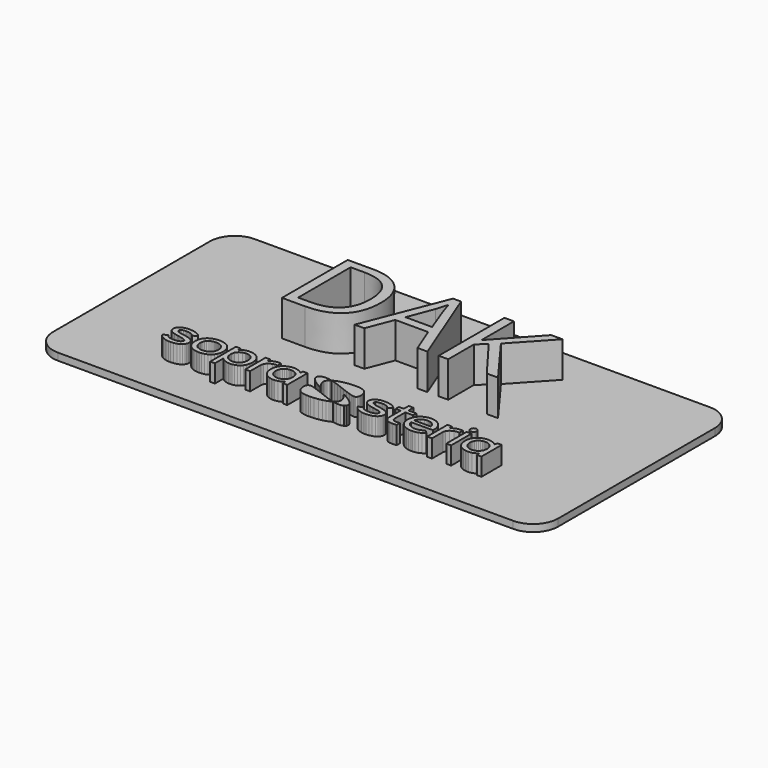
from build123d import *

# Parameters (mm, degrees)
F1_DEPTH     = 12.7
F0_W         = 3.439668
F0_H         = 17.9889404
F2_TEXT_SIZE = 81.8710528274
F3_DEPTH     = 25.4
F5_DEPTH     = 5.08


# Not quite as in the source:
# - Text() gives the source's letters only with a copy of the font that has no kerning and outlines rounded to 1/6400 em; it was checked with that copy


with BuildPart() as f1:
    # F0 (on Top) → F1 (new body)
    with BuildSketch(Plane.XY):
        Polygon((10.402189, -8.9867994), (10.078339, -9.2017596), (10.030333, -9.2320872), (9.500997, -9.561449), (9.448419, -9.5917512), (9.3881075175, -9.6273787491), (9.389237, -9.6275906), (9.38663303, -9.629093988), (9.448419, -9.6358456), (10.190099, -9.8384106), (12.472035, -10.2407974), (15.177135, -10.2821486), (17.257903, -9.6289622), (18.283047, -8.5747606), (18.410047, -8.1585816), (18.496915, -7.8691994), (18.455513, -6.9086222), (17.923637, -5.6614822), (16.941165, -4.4420282), (15.638653, -3.2733742), (14.143609, -2.1806662), (12.585065, -1.1885422), (11.092561, -0.3203702), (10.119741, 0.2186178), (9.795891, 0.3961638), (9.696577, 0.4500118), (9.375521, 0.5630418), (9.126093, 0.5409438), (9.080627, 0.3590798), (9.209913, 0.1152398), (9.269349, 0.0476758), (9.465183, -0.1783842), (10.023221, -0.8867902), (10.767441, -1.9794982), (11.413871, -3.1811722), (11.872341, -4.4460922), (12.055983, -5.7262522), (11.876659, -6.9777102), (11.246993, -8.1517236), align=None)
        Polygon((9.389237, -9.6275906), (9.3881075175, -9.6273787491), (9.385427, -9.6289622), (9.38663303, -9.629093988), align=None)
        Polygon((9.385427, -9.6289622), (9.3881075175, -9.6273787491), (8.749919, -9.5076772), (6.863461, -8.988171), (3.947541, -8.0138778), (0.805561, -6.8342002), (-2.398395, -5.5789322), (-5.497703, -4.3757342), (-8.328025, -3.3561782), (-10.724515, -2.6492962), (-12.073763, -2.3858982), (-12.522835, -2.3858982), (-12.767945, -2.3858982), (-13.502513, -2.6396442), (-14.194409, -3.3300162), (-14.606397, -4.3442382), (-14.741525, -5.2660042), (-14.741525, -5.5733442), (-14.741525, -5.9563762), (-14.609191, -7.1057262), (-14.216507, -8.6050628), (-13.575665, -9.9693222), (-12.948539, -10.8498894), (-12.695047, -11.0993174), (-12.437491, -11.3528856), (-11.446637, -11.8999762), (-9.662287, -12.4539502), (-7.450201, -12.7750062), (-5.552567, -12.8797558), (-4.918837, -12.8797558), (-4.109847, -12.8797558), (-1.681861, -12.7391922), (1.169543, -12.3712478), (3.620897, -11.8503446), (5.660263, -11.2536478), (7.269861, -10.6555794), (8.436991, -10.1347016), (9.148191, -9.7667572), (9.38663303, -9.629093988), align=None)
    extrude(amount=F1_DEPTH)


with BuildPart() as f1b:
    # F0 (on Top) → F1, piece 2 (new body)
    with BuildSketch(Plane.XY):
        Polygon((42.048811, 5.3156358), (45.511847, 5.3156358), (45.511847, -3.8108382), (45.511847, -4.0231822), (45.539533, -4.6640242), (45.657897, -5.6147462), (45.919771, -6.5959482), (46.377225, -7.5438762), (47.082837, -8.3956144), (48.087661, -9.0832686), (49.446053, -9.5435166), (50.768885, -9.7116138), (51.210083, -9.7116138), (51.641375, -9.7116138), (52.938299, -9.6454722), (54.256813, -9.4994222), (54.548913, -9.4608396), (54.548913, -6.4387222), (54.343681, -6.4857122), (53.813075, -6.5918842), (53.082825, -6.6965322), (52.477797, -6.7447922), (52.276883, -6.7447922), (51.848131, -6.7447922), (50.562383, -6.5311782), (49.521999, -5.8987182), (49.006633, -4.8568102), (48.868711, -3.7750242), (48.868711, -3.4153602), (48.868711, 5.3156358), (54.393465, 5.3156358), (54.393465, 8.2165698), (48.868711, 8.2165698), (48.868711, 12.5172978), (45.511847, 12.5172978), (45.511847, 8.2165698), (42.048811, 8.2165698), align=None)
    extrude(amount=F1_DEPTH)


with BuildPart() as f1c:
    # F0 (on Top) → F1, piece 3 (new body)
    with BuildSketch(Plane.XY):
        with Locations((91.832049, -0.7598664)):
            Rectangle(F0_W, F0_H)
    extrude(amount=F1_DEPTH)


with BuildPart() as f1d:
    # F0 (on Top) → F1, piece 4 (new body)
    with BuildSketch(Plane.XY):
        Polygon((96.128459, -0.0089662), (96.128459, -0.5918962), (96.128459, -1.1705082), (96.347661, -2.9096462), (96.963611, -4.8555402), (97.911793, -6.4471042), (99.127183, -7.7051916), (100.543741, -8.6491572), (102.096697, -9.2982288), (103.723059, -9.6730566), (104.947847, -9.7943162), (105.357041, -9.7943162), (106.061637, -9.7943162), (108.174155, -9.42086), (110.188883, -8.600948), (111.398431, -7.7810106), (111.802291, -7.4090022), (111.976027, -9.790176), (115.120547, -9.790176), (115.120547, 8.2330798), (111.981615, 8.2330798), (111.802291, 5.9966098), (111.406813, 6.3839598), (110.216315, 7.2340978), (108.216827, 8.0842358), (106.099991, 8.4703158), (105.395903, 8.4703158), (105.022269, 8.4703158), (103.906193, 8.3585558), (102.344855, 8.0057498), (100.793169, 7.3872598), (99.336733, 6.4759078), (98.057843, 5.2483258), (97.042097, 3.6788598), (96.369759, 1.7398238), align=None)
        Polygon((99.623499, -1.0437622), (99.623499, -0.6277102), (99.623499, -0.2045462), (99.799775, 1.0631678), (100.280597, 2.4246078), (100.995861, 3.4873438), (101.872415, 4.2838878), (102.835583, 4.8485298), (103.816531, 5.2112418), (104.741091, 5.4052978), (105.339515, 5.4616858), (105.539159, 5.4616858), (106.134535, 5.4616858), (107.923203, 5.1022758), (109.919897, 4.0011858), (111.292513, 2.1256498), (111.802291, 0.1137158), (111.802291, -0.5573522), (111.802291, -1.2340082), (111.342043, -3.2652462), (110.056549, -5.1999642), (108.087287, -6.3617602), (106.202099, -6.7488562), (105.575227, -6.7488562), (105.372281, -6.7488562), (104.768777, -6.6853562), (103.837359, -6.4813942), (102.850569, -6.1039502), (101.880543, -5.5250842), (101.001449, -4.7176182), (100.283391, -3.6510722), (99.799775, -2.2964902), align=None, mode=Mode.SUBTRACT)
    extrude(amount=F1_DEPTH)


with BuildPart() as f1e:
    # F0 (on Top) → F1, piece 5 (new body)
    with BuildSketch(Plane.XY):
        Polygon((94.080965, 12.1688098), (94.080965, 12.3864878), (94.080965, 12.6054358), (93.903165, 13.2630418), (93.420819, 13.9767818), (92.706825, 14.4591278), (92.049727, 14.6354038), (91.832049, 14.6354038), (91.612847, 14.6354038), (90.955241, 14.4591278), (90.241755, 13.9767818), (89.759409, 13.2630418), (89.583133, 12.6054358), (89.583133, 12.3864878), (89.583133, 12.1688098), (89.759409, 11.5114578), (90.241755, 10.7964478), (90.955241, 10.3153718), (91.612847, 10.1375718), (91.832049, 10.1375718), (92.049727, 10.1375718), (92.706825, 10.3153718), (93.420819, 10.7964478), (93.903165, 11.5114578), align=None)
    extrude(amount=F1_DEPTH)


with BuildPart() as f1f:
    # F0 (on Top) → F1, piece 6 (new body)
    with BuildSketch(Plane.XY):
        Polygon((86.724871, 5.1904138), (87.600155, 5.1406298), (87.600155, 8.1876138), (87.012653, 8.2412078), (85.235161, 8.2099658), (83.205193, 7.8101698), (81.461991, 6.9889878), (80.297655, 6.0943998), (79.964153, 5.7443878), (79.785083, 8.2252058), (76.524739, 8.2252058), (76.524739, -9.7777808), (79.964153, -9.7777808), (79.964153, -0.4499102), (79.964153, 0.0545338), (80.377665, 1.5663418), (81.704815, 3.4388298), (84.069555, 4.7647098), align=None)
    extrude(amount=F1_DEPTH)


with BuildPart() as f1g:
    # F0 (on Top) → F1, piece 7 (new body)
    with BuildSketch(Plane.XY):
        Polygon((55.218711, -0.1562862), (55.218711, -0.6607302), (55.218711, -0.7999222), (55.218711, -1.2903962), (55.409211, -2.7620722), (55.965725, -4.5245782), (56.861583, -6.0681362), (58.067321, -7.3716642), (59.556777, -8.4190586), (61.304043, -9.1907614), (63.281687, -9.6661478), (64.917447, -9.8301556), (65.463293, -9.8301556), (66.000503, -9.8301556), (67.612641, -9.6785684), (69.688075, -9.1659456), (71.684769, -8.204073), (73.162287, -7.1222362), (73.598913, -6.7046602), (71.139177, -4.5413422), (70.752081, -4.8857662), (69.636005, -5.6437022), (67.851147, -6.4016382), (66.058415, -6.7475862), (65.461769, -6.7475862), (64.856741, -6.7475862), (63.043181, -6.3754762), (60.941585, -5.3516022), (59.432825, -3.8067742), (58.820939, -2.3625302), (58.796047, -1.8733262), (74.168127, -1.8085562), (74.186161, -1.6350742), (74.231627, -0.8177022), (74.241025, -0.3493262), (74.241025, 0.0984758), (74.066019, 1.4408658), (73.562083, 3.1121858), (72.750299, 4.6295818), (71.655813, 5.9524138), (70.301231, 7.0468998), (68.713731, 7.8746858), (66.915665, 8.3986878), (65.427225, 8.5802978), (64.932687, 8.5802978), (64.428243, 8.5802978), (62.919483, 8.4151978), (61.071125, 7.9287878), (59.417839, 7.1416418), (57.991375, 6.0710318), (56.826785, 4.7372778), (55.954549, 3.1576518), (55.407687, 1.3527278), align=None)
        Polygon((70.465315, 1.1086338), (70.465315, 0.8840978), (58.848625, 0.8840978), (58.887233, 1.3318998), (59.442477, 2.6341578), (60.780549, 4.0590978), (62.685041, 5.0184558), (64.404875, 5.3682138), (64.979169, 5.3682138), (65.255013, 5.3682138), (66.083053, 5.2757578), (67.112515, 5.0126138), (68.044187, 4.5950378), (68.855971, 4.0438578), (69.526785, 3.3783778), (70.032753, 2.6176478), (70.352539, 1.7799558), align=None, mode=Mode.SUBTRACT)
    extrude(amount=F1_DEPTH)


with BuildPart() as f1h:
    # F0 (on Top) → F1, piece 8 (new body)
    with BuildSketch(Plane.XY):
        Polygon((35.330765, 0.8454898), (34.687383, 0.9597898), (34.053399, 1.0728198), (32.153225, 1.4103858), (29.956633, 1.9188938), (28.407487, 2.6148538), (27.821763, 3.3730438), (27.821763, 3.6247578), (27.821763, 3.8139878), (28.031313, 4.3773598), (28.721939, 5.0085498), (29.979747, 5.4413658), (31.415863, 5.6011318), (31.895415, 5.6011318), (32.323913, 5.6011318), (33.613725, 5.4949598), (35.252533, 5.1421538), (36.600003, 4.4891198), (37.320855, 3.7738558), (37.448871, 3.4845498), (40.640381, 4.8254158), (40.414575, 5.2800758), (39.305103, 6.4281558), (37.246433, 7.5622658), (34.639377, 8.2361278), (32.402653, 8.4578698), (31.656909, 8.4578698), (30.979237, 8.4578698), (28.949269, 8.1863438), (26.533475, 7.3128378), (24.797131, 5.7499758), (24.132921, 3.9955978), (24.132921, 3.4101278), (24.132921, 2.9084778), (24.659209, 1.4022578), (26.176605, 0.0199898), (28.589605, -0.9335262), (30.993969, -1.5055342), (31.802959, -1.6584422), (32.377761, -1.7658842), (34.105977, -2.0800822), (36.065333, -2.5512522), (37.425503, -3.2322262), (37.935281, -4.0203882), (37.935281, -4.2835322), (37.935281, -4.4943522), (37.651563, -5.1268122), (36.758499, -5.9276742), (35.187509, -6.5243202), (33.449641, -6.7585082), (32.871283, -6.7585082), (32.394271, -6.7585082), (30.966537, -6.6454782), (29.223589, -6.2596522), (27.815159, -5.5306722), (27.050365, -4.7120302), (26.910919, -4.3897042), (23.818977, -5.6876442), (24.047577, -6.1976762), (25.137491, -7.5507342), (27.098625, -8.8930734), (29.553027, -9.7047558), (31.654369, -9.977628), (32.355663, -9.977628), (33.014539, -9.977628), (34.990659, -9.8136202), (37.093525, -9.3643958), (38.719633, -8.6932516), (39.923847, -7.8609444), (40.763063, -6.9307202), (41.293669, -5.9619642), (41.570783, -5.0208942), (41.650793, -4.3800522), (41.650793, -4.1677082), (41.650793, -3.6193222), (41.051099, -1.9754342), (39.473505, -0.5228082), (37.242115, 0.3893058), align=None)
    extrude(amount=F1_DEPTH)


with BuildPart() as f1i:
    # F0 (on Top) → F1, piece 9 (new body)
    with BuildSketch(Plane.XY):
        Polygon((-64.928369, -9.7943162), (-64.221487, -9.7943162), (-63.813563, -9.7943162), (-62.588267, -9.690989), (-60.962413, -9.3574616), (-59.407679, -8.7607902), (-57.991375, -7.8650846), (-56.777001, -6.6345562), (-55.829073, -5.0346102), (-55.213123, -3.0323282), (-54.992651, -1.2007342), (-54.992651, -0.5918962), (-54.992651, 0.0171958), (-55.234967, 1.8447258), (-55.907559, 3.8315138), (-56.923051, 5.4080918), (-58.201941, 6.6125598), (-59.658631, 7.4822558), (-61.209047, 8.0568038), (-62.770385, 8.3735418), (-63.886715, 8.4703158), (-64.257047, 8.4703158), (-64.963929, 8.4703158), (-67.080511, 8.0842358), (-69.080253, 7.2340978), (-70.270751, 6.3839598), (-70.663689, 5.9966098), (-70.842759, 8.2330798), (-73.984739, 8.2330798), (-73.984739, -14.6353784), (-70.663689, -14.6353784), (-70.663689, -7.0561962), (-70.264147, -7.4834242), (-69.058409, -8.424545), (-67.046475, -9.3657674), align=None)
        Polygon((-64.997203, 5.4616858), (-64.400557, 5.4616858), (-64.201929, 5.4616858), (-63.604013, 5.4205378), (-62.679453, 5.2635658), (-61.699267, 4.9453038), (-60.734829, 4.4228258), (-59.860053, 3.6483798), (-59.144535, 2.5792938), (-58.663713, 1.1693398), (-58.485913, -0.1783842), (-58.485913, -0.6277102), (-58.485913, -1.0767822), (-58.663713, -2.4245062), (-59.147329, -3.8385242), (-59.865387, -4.9131982), (-60.744481, -5.6919622), (-61.713237, -6.2210442), (-62.699773, -6.5436242), (-63.631445, -6.7046602), (-64.235203, -6.7488562), (-64.436117, -6.7488562), (-65.066037, -6.7488562), (-66.951225, -6.3617602), (-68.920487, -5.1999642), (-70.204711, -3.2652462), (-70.663689, -1.2340082), (-70.663689, -0.5573522), (-70.663689, 0.1137158), (-70.155181, 2.1256498), (-68.782819, 4.0011858), (-66.787141, 5.1022758), align=None, mode=Mode.SUBTRACT)
    extrude(amount=F1_DEPTH)


with BuildPart() as f1j:
    # F0 (on Top) → F1, piece 10 (new body)
    with BuildSketch(Plane.XY):
        Polygon((-42.055669, -0.0089662), (-42.055669, -0.5918962), (-42.055669, -1.1705082), (-41.836467, -2.9096462), (-41.220517, -4.8555402), (-40.272335, -6.4471042), (-39.056945, -7.7051916), (-37.640387, -8.6491572), (-36.087431, -9.2982288), (-34.461069, -9.6730566), (-33.236281, -9.7943162), (-32.827087, -9.7943162), (-32.122745, -9.7943162), (-30.009973, -9.42086), (-27.995245, -8.600948), (-26.785697, -7.7810106), (-26.381837, -7.4090022), (-26.197179, -9.790176), (-23.063581, -9.790176), (-23.063581, 8.2330798), (-26.204037, 8.2330798), (-26.381837, 5.9966098), (-26.777315, 6.3839598), (-27.967813, 7.2340978), (-29.967301, 8.0842358), (-32.082613, 8.4703158), (-32.786701, 8.4703158), (-33.160335, 8.4703158), (-34.276411, 8.3585558), (-35.839273, 8.0057498), (-37.390959, 7.3872598), (-38.847395, 6.4759078), (-40.126285, 5.2483258), (-41.142031, 3.6788598), (-41.814369, 1.7398238), align=None)
        Polygon((-38.561137, -1.0437622), (-38.561137, -0.6277102), (-38.561137, -0.2045462), (-38.384607, 1.0631678), (-37.903531, 2.4246078), (-37.188267, 3.4873438), (-36.311967, 4.2838878), (-35.348545, 4.8485298), (-34.367597, 5.2112418), (-33.443037, 5.4052978), (-32.844613, 5.4616858), (-32.644969, 5.4616858), (-32.049847, 5.4616858), (-30.260925, 5.1022758), (-28.264231, 4.0011858), (-26.891615, 2.1256498), (-26.381837, 0.1137158), (-26.381837, -0.5573522), (-26.381837, -1.2340082), (-26.842085, -3.2652462), (-28.127579, -5.1999642), (-30.096841, -6.3617602), (-31.982029, -6.7488562), (-32.608901, -6.7488562), (-32.811847, -6.7488562), (-33.415351, -6.6853562), (-34.348039, -6.4813942), (-35.334829, -6.1039502), (-36.303585, -5.5250842), (-37.182679, -4.7176182), (-37.900737, -3.6510722), (-38.384607, -2.2964902), align=None, mode=Mode.SUBTRACT)
    extrude(amount=F1_DEPTH)


with BuildPart() as f1k:
    # F0 (on Top) → F1, piece 11 (new body)
    with BuildSketch(Plane.XY):
        Polygon((-42.679747, 5.1904138), (-41.804717, 5.1406298), (-41.804717, 8.1876138), (-42.391711, 8.2412078), (-44.169457, 8.2099658), (-46.200695, 7.8101698), (-47.942373, 6.9889878), (-49.106963, 6.0943998), (-49.440211, 5.7443878), (-49.618011, 8.2252058), (-52.881403, 8.2252058), (-52.881403, -9.7777808), (-49.440211, -9.7777808), (-49.440211, -0.4499102), (-49.440211, 0.0545338), (-49.027207, 1.5663418), (-47.700057, 3.4388298), (-45.335317, 4.7647098), align=None)
    extrude(amount=F1_DEPTH)


with BuildPart() as f1l:
    # F0 (on Top) → F1, piece 12 (new body)
    with BuildSketch(Plane.XY):
        Polygon((-103.608505, 0.8454898), (-104.251887, 0.9597898), (-104.885871, 1.0728198), (-106.786045, 1.4103858), (-108.982764, 1.9188938), (-110.5303098, 2.6148538), (-111.115983, 3.3730438), (-111.115983, 3.6247578), (-111.115983, 3.8139878), (-110.9065092, 4.3773598), (-110.2161118, 5.0085498), (-108.9579736, 5.4413658), (-107.522137, 5.6011318), (-107.042585, 5.6011318), (-106.613833, 5.6011318), (-105.324021, 5.4949598), (-103.685721, 5.1421538), (-102.337743, 4.4891198), (-101.617145, 3.7738558), (-101.490399, 3.4845498), (-98.297365, 4.8254158), (-98.523425, 5.2800758), (-99.632897, 6.4281558), (-101.691567, 7.5622658), (-104.298877, 8.2361278), (-106.535347, 8.4578698), (-107.280837, 8.4578698), (-107.9588646, 8.4578698), (-109.9887056, 8.1863438), (-112.4058204, 7.3128378), (-114.142139, 5.7499758), (-114.806349, 3.9955978), (-114.806349, 3.4101278), (-114.806349, 2.9084778), (-114.279934, 1.4022578), (-112.7613442, 0.0199898), (-110.3484204, -0.9335262), (-107.9437262, -1.5055342), (-107.134787, -1.6584422), (-106.560239, -1.7658842), (-104.832023, -2.0800822), (-102.872667, -2.5512522), (-101.512497, -3.2322262), (-101.001195, -4.0203882), (-101.001195, -4.2835322), (-101.001195, -4.4943522), (-101.285167, -5.1268122), (-102.177977, -5.9276742), (-103.750491, -6.5243202), (-105.488105, -6.7585082), (-106.066971, -6.7585082), (-106.543729, -6.7585082), (-107.9726568, -6.6454782), (-109.7145126, -6.2596522), (-111.1228664, -5.5306722), (-111.8876858, -4.7120302), (-112.0268524, -4.3897042), (-115.120547, -5.6876442), (-114.8917946, -6.1976762), (-113.8017536, -7.5507342), (-111.8407974, -8.8930734), (-109.3851508, -9.7047558), (-107.285155, -9.977628), (-106.583607, -9.977628), (-105.924985, -9.977628), (-103.948865, -9.8136202), (-101.845999, -9.3643958), (-100.219891, -8.6932516), (-99.015423, -7.8609444), (-98.174937, -6.9307202), (-97.645601, -5.9619642), (-97.368741, -5.0208942), (-97.287207, -4.3800522), (-97.287207, -4.1677082), (-97.287207, -3.6193222), (-97.886901, -1.9754342), (-99.466019, -0.5228082), (-101.697155, 0.3893058), align=None)
    extrude(amount=F1_DEPTH)


with BuildPart() as f1m:
    # F0 (on Top) → F1, piece 13 (new body)
    with BuildSketch(Plane.XY):
        Polygon((-85.429217, 8.4703158), (-85.866097, 8.4703158), (-86.304501, 8.4703158), (-87.618951, 8.3585558), (-89.377139, 8.0057498), (-91.067001, 7.3872598), (-92.615639, 6.4759078), (-93.947107, 5.2483258), (-94.990285, 3.6788598), (-95.669481, 1.7398238), (-95.912051, -0.0089662), (-95.912051, -0.5918962), (-95.912051, -1.1720322), (-95.691579, -2.9137102), (-95.067247, -4.8705262), (-94.091887, -6.4788542), (-92.819601, -7.7548486), (-91.306523, -8.7166958), (-89.607517, -9.3823028), (-87.775923, -9.7681288), (-86.344379, -9.893554), (-85.866097, -9.893554), (-85.389339, -9.893554), (-83.957541, -9.7681288), (-82.126201, -9.3823028), (-80.426941, -8.7166958), (-78.915387, -7.7548486), (-77.643609, -6.4788542), (-76.667741, -4.8705262), (-76.043663, -2.9137102), (-75.821667, -1.1720322), (-75.821667, -0.5918962), (-75.821667, -0.0089662), (-76.065507, 1.7398238), (-76.744957, 3.6788598), (-77.788135, 5.2483258), (-79.119095, 6.4759078), (-80.666717, 7.3872598), (-82.356325, 8.0057498), (-84.114513, 8.3585558), align=None)
        Polygon((-85.313647, -6.7488562), (-85.866097, -6.7488562), (-86.421595, -6.7488562), (-88.083263, -6.4813942), (-90.201369, -5.5250842), (-91.790139, -3.6510722), (-92.415995, -1.3828522), (-92.415995, -0.6277102), (-92.415995, -0.2058162), (-92.234131, 1.0591038), (-91.733751, 2.4080978), (-90.982673, 3.4555938), (-90.049985, 4.2341038), (-89.002489, 4.7799498), (-87.911051, 5.1256438), (-86.843235, 5.3090318), (-86.111715, 5.3613558), (-85.866097, 5.3613558), (-85.622257, 5.3613558), (-84.890737, 5.3090318), (-83.822413, 5.1256438), (-82.731229, 4.7799498), (-81.683987, 4.2341038), (-80.750791, 3.4555938), (-79.999713, 2.4080978), (-79.499587, 1.0591038), (-79.316453, -0.2058162), (-79.316453, -0.6277102), (-79.316453, -1.3828522), (-79.943325, -3.6510722), (-81.532095, -5.5250842), (-83.651725, -6.4813942), align=None, mode=Mode.SUBTRACT)
    extrude(amount=F1_DEPTH)


with BuildPart() as f1n:
    # F0 (on Top) → F1, piece 14 (new body)
    with BuildSketch(Plane.XY):
        Polygon((-8.180451, 9.0189558), (-7.856601, 9.2323158), (-7.810119, 9.2640658), (-7.279513, 9.5932498), (-7.226935, 9.6222058), (-7.1666285104, 9.6578084264), (-7.167753, 9.6580198), (-7.1648908296, 9.659698252), (-7.226935, 9.6676718), (-7.969885, 9.8713798), (-10.251567, 10.2739698), (-12.956667, 10.3138478), (-15.037689, 9.6608138), (-16.061563, 8.6067138), (-16.188563, 8.1891378), (-16.276701, 7.9011018), (-16.235045, 6.9407278), (-15.703423, 5.6935878), (-14.720697, 4.4738798), (-13.417169, 3.3052258), (-11.923395, 2.2127718), (-10.364851, 1.2203938), (-8.872347, 0.3522218), (-7.899781, -0.1865122), (-7.574407, -0.3658362), (-7.476363, -0.4194302), (-7.154037, -0.5311902), (-6.905879, -0.5090922), (-6.860413, -0.3272282), (-6.989953, -0.0833882), (-7.047865, -0.0170942), (-7.244969, 0.2102358), (-7.803007, 0.9186418), (-8.546973, 2.0113498), (-9.193403, 3.2127698), (-9.652381, 4.4779438), (-9.835769, 5.7581038), (-9.656445, 7.0093078), (-9.026779, 8.1835498), align=None)
        Polygon((-7.167753, 9.6580198), (-7.1666285104, 9.6578084264), (-7.163689, 9.6595438), (-7.1648908296, 9.659698252), align=None)
        Polygon((-7.163689, 9.6595438), (-7.1666285104, 9.6578084264), (-6.529959, 9.5381318), (-4.643247, 9.0199718), (-1.727073, 8.0458818), (1.414653, 6.8660518), (4.618609, 5.6092598), (7.717663, 4.4075858), (10.548239, 3.3880298), (12.945999, 2.6811478), (14.293977, 2.4164798), (14.744319, 2.4164798), (14.988159, 2.4164798), (15.722727, 2.6712418), (16.415893, 3.3616138), (16.827881, 4.3758358), (16.964533, 5.2981098), (16.964533, 5.6039258), (16.964533, 5.9884818), (16.830675, 7.1375778), (16.437991, 8.6356698), (15.795625, 10.0014278), (15.168753, 10.8817918), (14.916531, 11.1299498), (14.657705, 11.3849658), (13.666597, 11.9318278), (11.882247, 12.4860558), (9.670415, 12.8068578), (7.772781, 12.9102358), (7.140321, 12.9102358), (6.330061, 12.9102358), (3.902075, 12.7710438), (1.050925, 12.4029978), (-1.400937, 11.8822978), (-3.438779, 11.2841278), (-5.049647, 10.6874818), (-6.217031, 10.1665278), (-6.928231, 9.7984818), (-7.1648908296, 9.659698252), align=None)
    extrude(amount=F1_DEPTH)


with BuildPart() as f3:
    # F2 (on Top) → F3 (new body)
    with BuildSketch(Plane.XY):
        with Locations((-83.527662412, 51.1035351186)):
            Text('DAK', F2_TEXT_SIZE, font='Open Sans', text_align=(TextAlign.LEFT, TextAlign.BOTTOM))
    extrude(amount=F3_DEPTH)


with BuildPart() as f5:
    # F4 (on Top) → F5 (new body)
    with BuildSketch(Plane.XY):
        with BuildLine():
            Line((161.9547217798, 134.9517914262), (-161.9547217798, 134.9517914262))
            ThreePointArc((-161.9547217798, 134.9517914262), (-174.5270803493, 129.7441499957), (-179.7347217798, 117.1717914262))
            Line((-179.7347217798, 117.1717914262), (-179.7347217798, -22.2553784))
            ThreePointArc((-179.7347217798, -22.2553784), (-174.5270803493, -34.8277369695), (-161.9547217798, -40.0353784))
            Line((-161.9547217798, -40.0353784), (161.9547217798, -40.0353784))
            ThreePointArc((161.9547217798, -40.0353784), (174.5270803493, -34.8277369695), (179.7347217798, -22.2553784))
            Line((179.7347217798, -22.2553784), (179.7347217798, 117.1717914262))
            ThreePointArc((179.7347217798, 117.1717914262), (174.5270803493, 129.7441499957), (161.9547217798, 134.9517914262))
        make_face()
    extrude(amount=-F5_DEPTH)


solid = Compound([f1.part, f1b.part, f1c.part, f1d.part, f1e.part, f1f.part, f1g.part, f1h.part, f1i.part, f1j.part, f1k.part, f1l.part, f1m.part, f1n.part, f3.part, f5.part])
